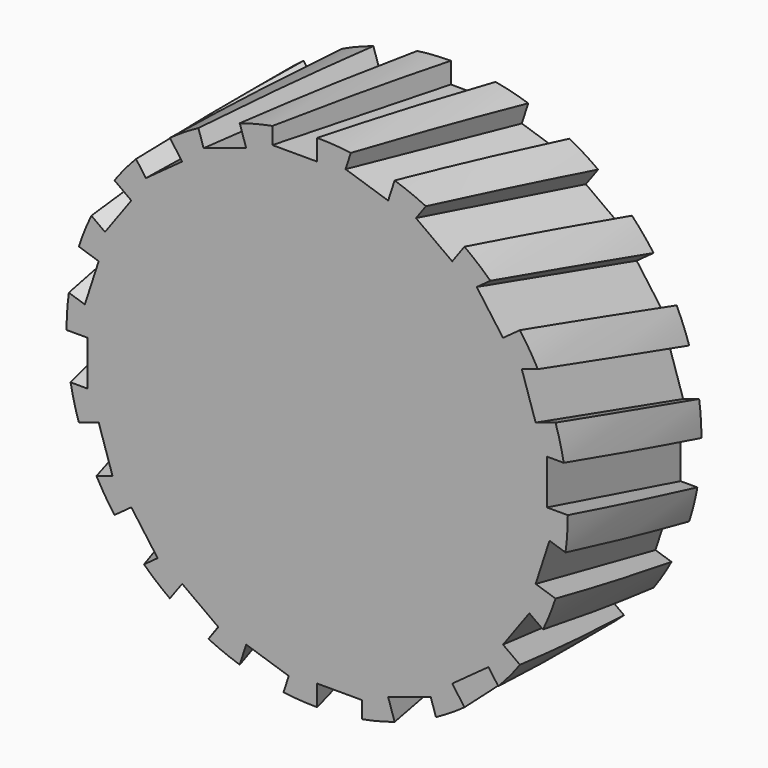
from build123d import *

# Parameters (mm, degrees)
F0_R            = 38.1
F1_DEPTH        = 12.7
F4_DEPTH        = 3.175
F4_COPIES_COUNT = 20


# Not quite as in the source:
# - a pattern or mirror of a feature is missing from the dataset's text; its kind, count and spacing are read off the source's solid


with BuildPart() as f1:
    # F0 (on Front) → F1 (new body, symmetric)
    with BuildSketch(Plane.XZ):
        Circle(F0_R)
    extrude(amount=F1_DEPTH, both=True)

    # F3 (on offset) → F4 (cut)
    with BuildSketch(Plane.XY.offset(38.1)):
        Polygon((-6.8059094878, -12.7), (0, -12.7), (6.8059094878, 12.7), (0, 12.7), align=None)
    f4 = extrude(amount=-F4_DEPTH, mode=Mode.SUBTRACT)

    # F4_copies: F4 ×20 about axis
    f4_copies_axis = Axis((0, 0, 0), (0, 1, 0))
    for i in range(1, F4_COPIES_COUNT):
        add(f4.rotate(f4_copies_axis, i * 360 / F4_COPIES_COUNT), mode=Mode.SUBTRACT)


solid = f1.part
